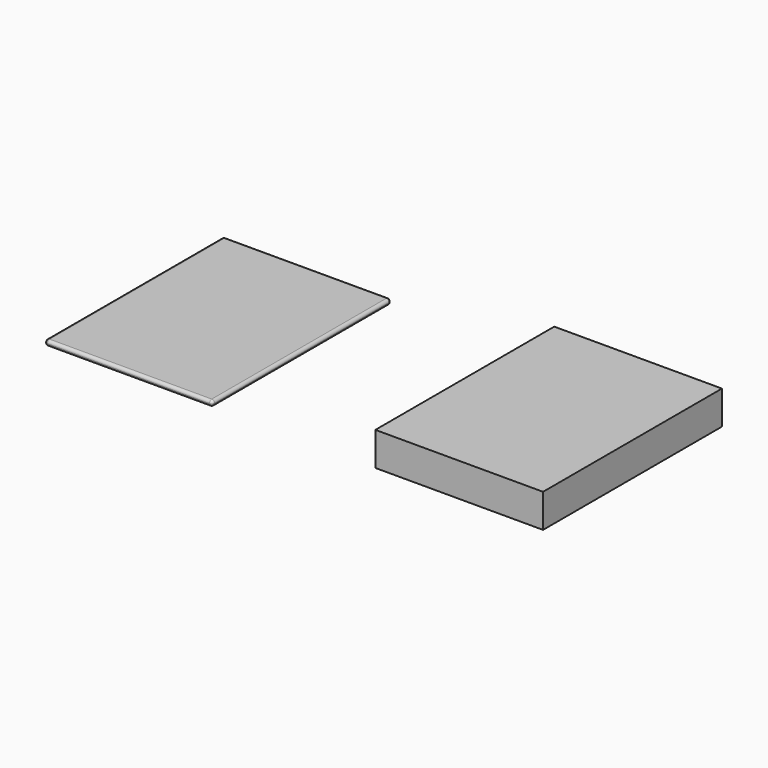
from build123d import *

# Parameters (mm, degrees)
F0_W     = 1524
F0_H     = 2032
F1_DEPTH = 304.8
F2_W     = 1524
F2_H     = 2032
F3_DEPTH = 50.8
F4_R     = 25.39999


# Not quite as in the source:
# - a fillet or chamfer is up to 0.001 mm smaller than in the source, because OpenCascade refuses the exact size


with BuildPart() as f1:
    # F0 (on Top) → F1 (new body)
    with BuildSketch(Plane.XY):
        Rectangle(F0_W, F0_H)
    extrude(amount=F1_DEPTH)


with BuildPart() as f3:
    # F2 (on Top) → F3 (new body)
    with BuildSketch(Plane.XY):
        with Locations((-3005.7537959279, 0)):
            Rectangle(F2_W, F2_H)
    extrude(amount=F3_DEPTH)

    # F4 (radius 25.4 in the source; OpenCascade refuses exactly that, so slightly less here)
    f4_edges = [f3.edges().sort_by_distance(p)[0] for p in [
        (-2243.753796, 0, 50.8),
        (-2243.753796, 0, 0),
        (-2243.753796, -1016, 25.4),
        (-3005.753796, -1016, 50.8),
        (-3767.753796, 0, 50.8),
        (-3767.753796, -1016, 25.4),
        (-3005.753796, -1016, 0),
        (-3767.753796, 0, 0),
        (-3767.753796, 1016, 25.4),
        (-3005.753796, 1016, 0),
        (-3005.753796, 1016, 50.8),
        (-2243.753796, 1016, 25.4),
    ]]
    fillet(f4_edges, radius=F4_R)


solid = Compound([f1.part, f3.part])
